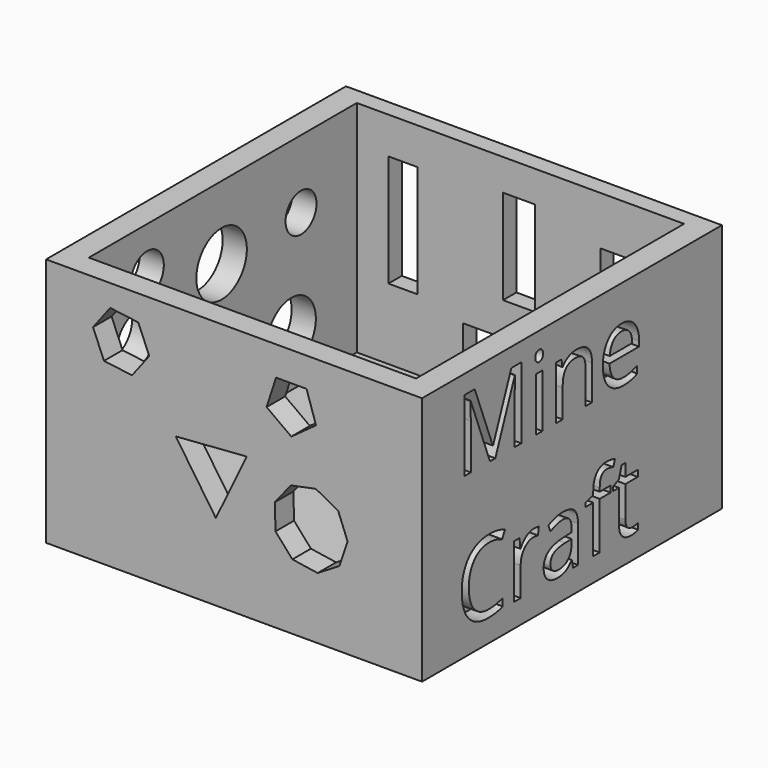
from build123d import *

# Parameters (mm, degrees)
F0_W          = 150.6570279598
F0_H          = 150.2079218626
F1_DEPTH      = 100
F3_W          = 131.1331391335
F3_H          = 134.2289075255
F4_DEPTH      = 88
F6_DEPTH      = 25
F7_R          = 12.6561324636
F7_R_2        = 12.3317055465
F7_R_3        = 8.1095155377
F7_R_4        = 9.8852980551
F7_R_5        = 9.1989445907
F7_R_6        = 7.7497110036
F7_R_7        = 8.3179289501
F8_DEPTH      = 25
F9_W          = 11.7512196302
F9_H          = 44.8682233691
F9_W_2        = 37.9243157804
F9_H_2        = 14.9560719728
F9_W_3        = 12.8194871359
F9_H_3        = 37.924323231
F9_W_4        = 17.0926488936
F9_H_4        = 32.0487245917
F9_W_5        = 19.7633728385
F9_H_5        = 19.7633802891
F10_DEPTH     = 25
F11_TEXT_SIZE = 40.0609129833
F12_DEPTH     = 8


# Not quite as in the source:
# - Text() gives the source's letters only with a copy of the font that has no kerning and outlines rounded to 1/6400 em; it was checked with that copy


with BuildPart() as f1:
    # F0 (on Top) → F1 (new body)
    with BuildSketch(Plane.XY):
        with Locations((1.1084377766, -0.6695911288)):
            Rectangle(F0_W, F0_H)
    extrude(amount=F1_DEPTH)

    # F3 (on face) → F4 (cut)
    with BuildSketch(Plane.XY.offset(100)):
        with Locations((1.051299274, 0.6259568036)):
            Rectangle(F3_W, F3_H)
    extrude(amount=-F4_DEPTH, mode=Mode.SUBTRACT)

    # F5 (on face) → F6 (cut)
    with BuildSketch(Plane.XZ.offset(75.7735520601)):
        Polygon((30.1584928658, 88.2577449083), (17.9330900881, 88.2577449083), (14.1552328667, 76.6306959322), (24.045791477, 69.4447844761), (33.9363500872, 76.6306959322), align=None)
        Polygon((42.8598879911, 49.2960034629), (33.8734404109, 54.1923673133), (23.8421001632, 52.1668224728), (17.4596428357, 44.1671438836), (17.7124911451, 33.9364700642), (24.4823345574, 26.2618469959), (34.6014881015, 24.7343161063), (43.3350873722, 30.0686260753), (46.5965842077, 39.7687939841), align=None)
        Polygon((-48.5306992416, 91.2351571948), (-55.4035291787, 82.2053140967), (-51.0198706321, 71.7383472262), (-39.7633821484, 70.3012234538), (-32.8905522112, 79.3310665519), (-37.2742107578, 89.7980334224), align=None)
        Polygon((-6.191431525, 30.8894089294), (6.191431525, 56.5846392083), (-22.2527221777, 54.4608980417), align=None)
    extrude(amount=-F6_DEPTH, mode=Mode.SUBTRACT)

    # F7 (on face) → F8 (cut)
    with BuildSketch(Plane(origin=(-74.2200762033, 0, 0), x_dir=(0, -1, 0), z_dir=(-1, 0, 0))):
        with Locations((0, 70.7963481545)):
            Circle(F7_R)
        with Locations((-34.8874144256, 32.2711616755)):
            Circle(F7_R_2)
        with Locations((42.5406396389, 33.4042571485)):
            Circle(F7_R_3)
        with Locations((42.5406396389, 61.3538958132)):
            Circle(F7_R_4)
        with Locations((0, 43.6020977795)):
            Circle(F7_R_5)
        with Locations((-39.7974848747, 72.6848319173)):
            Circle(F7_R_6)
        with Locations((37.2528731823, 82.1272805333)):
            Circle(F7_R_7)
    extrude(amount=-F8_DEPTH, mode=Mode.SUBTRACT)

    # F9 (on face) → F10 (cut)
    with BuildSketch(Plane(origin=(0, 74.4343698025, 0), x_dir=(-1, 0, 0), z_dir=(0, 1, 0))):
        with Locations((45.9755919874, 62.8335289657)):
            Rectangle(F9_W, F9_H)
        with Locations((2.9768869281, 28.6482200027)):
            Rectangle(F9_W_2, F9_H_2)
        with Locations((-0.4950582515, 68.4420522302)):
            Rectangle(F9_W_3, F9_H_3)
        with Locations((-34.1462213546, 33.4555283189)):
            Rectangle(F9_W_4, F9_H_4)
        with Locations((-42.9596193135, 70.5786347389)):
            Rectangle(F9_W_5, F9_H_5)
    extrude(amount=-F10_DEPTH, mode=Mode.SUBTRACT)

    # F11 (on face) → F12 (cut)
    with BuildSketch(Plane.YZ.offset(76.4369517565)):
        with Locations((-58.3351282403, 63.8935640454)):
            Text('Mine', F11_TEXT_SIZE, font='Open Sans', text_align=(TextAlign.LEFT, TextAlign.BOTTOM))
        with Locations((-58.3351282403, 9.4107223882)):
            Text('Craft', F11_TEXT_SIZE, font='Open Sans', text_align=(TextAlign.LEFT, TextAlign.BOTTOM))
    extrude(amount=-F12_DEPTH, mode=Mode.SUBTRACT)


solid = f1.part
